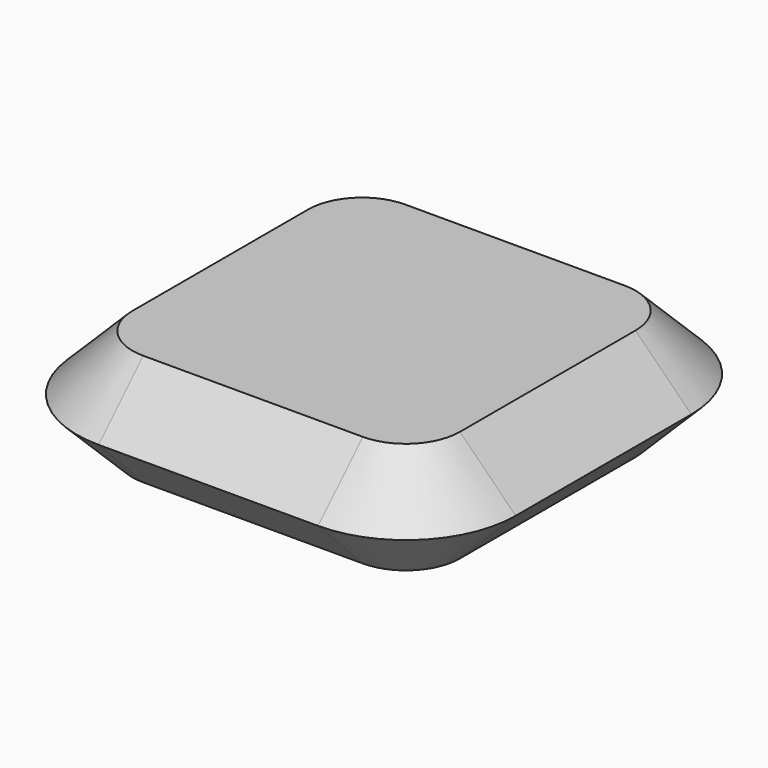
from build123d import *

# Parameters (mm, degrees)
F1_DEPTH = 25.4
F2_SIZE  = 12.69999


# Not quite as in the source:
# - a fillet or chamfer is up to 0.001 mm smaller than in the source, because OpenCascade refuses the exact size


with BuildPart() as f1:
    # F0 (on Top) → F1 (new body)
    with BuildSketch(Plane.XY):
        with BuildLine():
            ThreePointArc((50, 25), (42.6776695297, 42.6776695297), (25, 50))
            Line((25, 50), (-25, 50))
            ThreePointArc((-25, 50), (-42.6776695297, 42.6776695297), (-50, 25))
            Line((-50, 25), (-50, -25))
            ThreePointArc((-50, -25), (-42.6776695297, -42.6776695297), (-25, -50))
            Line((-25, -50), (25, -50))
            ThreePointArc((25, -50), (42.6776695297, -42.6776695297), (50, -25))
            Line((50, -25), (50, 25))
        make_face()
    extrude(amount=F1_DEPTH)

    # F2 (size 12.7 in the source; OpenCascade refuses exactly that, so slightly less here)
    f2_edges = [f1.edges().sort_by_distance(p)[0] for p in [
        (42.67767, 42.67767, 25.4),
        (0, 50, 25.4),
        (-42.67767, 42.67767, 25.4),
        (-50, 0, 25.4),
        (-42.67767, -42.67767, 25.4),
        (0, -50, 25.4),
        (42.67767, -42.67767, 25.4),
        (50, 0, 25.4),
        (42.67767, 42.67767, 0),
        (0, 50, 0),
        (-42.67767, 42.67767, 0),
        (-50, 0, 0),
        (-42.67767, -42.67767, 0),
        (0, -50, 0),
        (42.67767, -42.67767, 0),
        (50, 0, 0),
    ]]
    chamfer(f2_edges, length=F2_SIZE)


solid = f1.part
